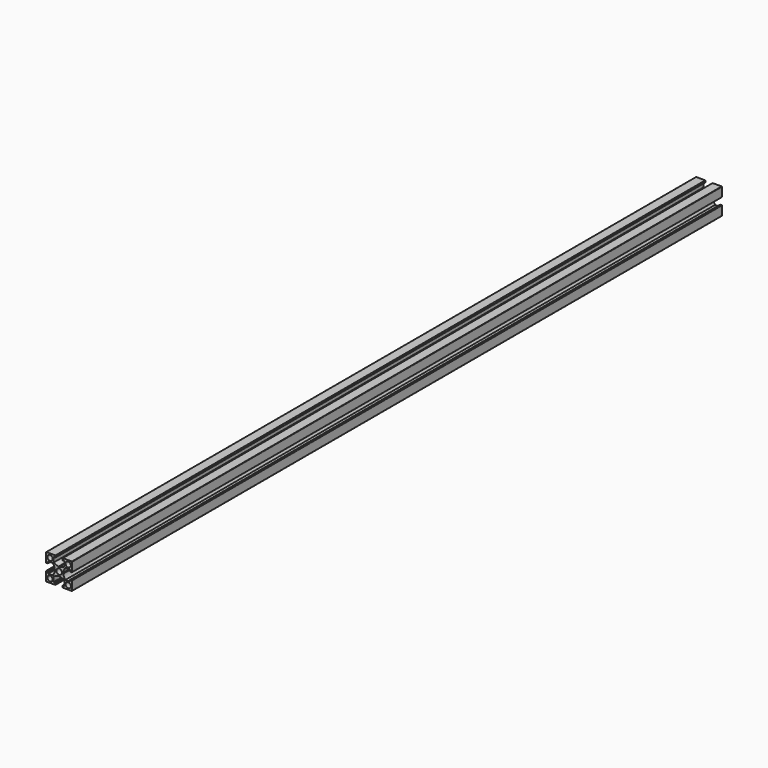
from build123d import *

# Parameters (mm, degrees)
F0_R     = 2
F0_R_2   = 2.15
F1_DEPTH = 312


# Not quite as in the source:
# - ends of sketch curves that miss each other by under 0.0002 mm in the source are joined


with BuildPart() as f1:
    # F0 (on Front) → F1 (new body, symmetric)
    with BuildSketch(Plane.XZ):
        with BuildLine():
            Line((4.49119, 14.509531), (4.49119, 11.252281))
            ThreePointArc((4.49119, 11.252281), (4.4613472004, 11.1218391084), (4.377756086, 11.0173488916))
            ThreePointArc((4.377756086, 11.0173488916), (2.6232116259, 10.0239112371), (0.6484679813, 9.6168093955))
            Line((0.6484679813, 9.6168093955), (0.34119, 9.309531))
            Line((0.34119, 9.309531), (0.033913, 9.616809))
            ThreePointArc((0.033913, 9.616809), (-1.9408311583, 10.0239110615), (-3.695375823, 11.0173492229))
            ThreePointArc((-3.695375823, 11.0173492229), (-3.7789672004, 11.1218391084), (-3.80881, 11.252281))
            Line((-3.80881, 11.252281), (-3.80881, 14.509531))
            ThreePointArc((-3.80881, 14.509531), (-3.7209420344, 14.7216630344), (-3.50881, 14.809531))
            Line((-3.50881, 14.809531), (-2.60881, 14.809531))
            ThreePointArc((-2.60881, 14.809531), (-2.3966779656, 14.8973989656), (-2.30881, 15.109531))
            Line((-2.30881, 15.109531), (-2.30881, 16.009531))
            ThreePointArc((-2.30881, 16.009531), (-2.3966779656, 16.2216630344), (-2.60881, 16.309531))
            Line((-2.60881, 16.309531), (-9.35881, 16.309531))
            ThreePointArc((-9.35881, 16.309531), (-9.5709420344, 16.2216630344), (-9.65881, 16.009531))
            Line((-9.65881, 16.009531), (-9.65881, 9.259531))
            ThreePointArc((-9.65881, 9.259531), (-9.5709420344, 9.0473989656), (-9.35881, 8.959531))
            Line((-9.35881, 8.959531), (-8.45881, 8.959531))
            ThreePointArc((-8.45881, 8.959531), (-8.2466779656, 9.0473989656), (-8.15881, 9.259531))
            Line((-8.15881, 9.259531), (-8.15881, 10.159531))
            ThreePointArc((-8.15881, 10.159531), (-8.0709420344, 10.3716630344), (-7.85881, 10.459531))
            Line((-7.85881, 10.459531), (-4.601559, 10.459531))
            ThreePointArc((-4.601559, 10.459531), (-4.471117461, 10.4296883706), (-4.3666273786, 10.3460976993))
            ThreePointArc((-4.3666273786, 10.3460976993), (-3.3731893747, 8.5915529924), (-2.9660873955, 6.6168089813))
            Line((-2.9660873955, 6.6168089813), (-2.65881, 6.309531))
            Line((-2.65881, 6.309531), (-2.966087, 6.002254))
            ThreePointArc((-2.966087, 6.002254), (-3.3731890615, 4.0275098417), (-4.3666272229, 2.272965177))
            ThreePointArc((-4.3666272229, 2.272965177), (-4.4711171084, 2.1893737996), (-4.601559, 2.159531))
            Line((-4.601559, 2.159531), (-7.85881, 2.159531))
            ThreePointArc((-7.85881, 2.159531), (-8.0709420344, 2.2473989656), (-8.15881, 2.459531))
            Line((-8.15881, 2.459531), (-8.15881, 3.359531))
            ThreePointArc((-8.15881, 3.359531), (-8.2466779656, 3.5716630344), (-8.45881, 3.659531))
            Line((-8.45881, 3.659531), (-9.35881, 3.659531))
            ThreePointArc((-9.35881, 3.659531), (-9.5709420344, 3.5716630344), (-9.65881, 3.359531))
            Line((-9.65881, 3.359531), (-9.65881, -3.390469))
            ThreePointArc((-9.65881, -3.390469), (-9.5709420344, -3.6026010344), (-9.35881, -3.690469))
            Line((-9.35881, -3.690469), (-2.60881, -3.690469))
            ThreePointArc((-2.60881, -3.690469), (-2.3966779656, -3.6026010344), (-2.30881, -3.390469))
            Line((-2.30881, -3.390469), (-2.30881, -2.490469))
            ThreePointArc((-2.30881, -2.490469), (-2.3966779656, -2.2783369656), (-2.60881, -2.190469))
            Line((-2.60881, -2.190469), (-3.50881, -2.190469))
            ThreePointArc((-3.50881, -2.190469), (-3.7209420344, -2.1026010344), (-3.80881, -1.890469))
            Line((-3.80881, -1.890469), (-3.80881, 1.366782))
            ThreePointArc((-3.80881, 1.366782), (-3.7789672004, 1.4972238916), (-3.695376086, 1.6017141084))
            ThreePointArc((-3.695376086, 1.6017141084), (-1.9408311583, 2.5951519385), (0.0339130165, 3.0022536517))
            Line((0.0339130165, 3.0022536517), (0.34119, 3.309531))
            Line((0.34119, 3.309531), (0.648468, 3.002254))
            ThreePointArc((0.648468, 3.002254), (2.6232116259, 2.5951517629), (4.377755823, 1.6017137771))
            ThreePointArc((4.377755823, 1.6017137771), (4.4613472004, 1.4972238916), (4.49119, 1.366782))
            Line((4.49119, 1.366782), (4.49119, -1.890469))
            ThreePointArc((4.49119, -1.890469), (4.4033220344, -2.1026010344), (4.19119, -2.190469))
            Line((4.19119, -2.190469), (3.29119, -2.190469))
            ThreePointArc((3.29119, -2.190469), (3.0790579656, -2.2783369656), (2.99119, -2.490469))
            Line((2.99119, -2.490469), (2.99119, -3.390469))
            ThreePointArc((2.99119, -3.390469), (3.0790579656, -3.6026010344), (3.29119, -3.690469))
            Line((3.29119, -3.690469), (10.04119, -3.690469))
            ThreePointArc((10.04119, -3.690469), (10.2533220344, -3.6026010344), (10.34119, -3.390469))
            Line((10.34119, -3.390469), (10.34119, 3.359531))
            ThreePointArc((10.34119, 3.359531), (10.2533220344, 3.5716630344), (10.04119, 3.659531))
            Line((10.04119, 3.659531), (9.14119, 3.659531))
            ThreePointArc((9.14119, 3.659531), (8.9290579656, 3.5716630344), (8.84119, 3.359531))
            Line((8.84119, 3.359531), (8.84119, 2.459531))
            ThreePointArc((8.84119, 2.459531), (8.7533220344, 2.2473989656), (8.54119, 2.159531))
            Line((8.54119, 2.159531), (5.28394, 2.159531))
            ThreePointArc((5.28394, 2.159531), (5.1534981084, 2.1893737996), (5.0490078916, 2.272964914))
            ThreePointArc((5.0490078916, 2.272964914), (4.0555700615, 4.0275098417), (3.6484683483, 6.0022540165))
            Line((3.6484683483, 6.0022540165), (3.34119, 6.309531))
            Line((3.34119, 6.309531), (3.648468, 6.616809))
            ThreePointArc((3.648468, 6.616809), (4.0555703747, 8.5915529924), (5.0490087099, 10.3460974363))
            ThreePointArc((5.0490087099, 10.3460974363), (5.153498461, 10.4296883706), (5.28394, 10.459531))
            Line((5.28394, 10.459531), (8.54119, 10.459531))
            ThreePointArc((8.54119, 10.459531), (8.7533220344, 10.3716630344), (8.84119, 10.159531))
            Line((8.84119, 10.159531), (8.84119, 9.259531))
            ThreePointArc((8.84119, 9.259531), (8.9290579656, 9.0473989656), (9.14119, 8.959531))
            Line((9.14119, 8.959531), (10.04119, 8.959531))
            ThreePointArc((10.04119, 8.959531), (10.2533220344, 9.0473989656), (10.34119, 9.259531))
            Line((10.34119, 9.259531), (10.34119, 16.009531))
            ThreePointArc((10.34119, 16.009531), (10.2533220344, 16.2216630344), (10.04119, 16.309531))
            Line((10.04119, 16.309531), (3.29119, 16.309531))
            ThreePointArc((3.29119, 16.309531), (3.0790579656, 16.2216630344), (2.99119, 16.009531))
            Line((2.99119, 16.009531), (2.99119, 15.109531))
            ThreePointArc((2.99119, 15.109531), (3.0790579656, 14.8973989656), (3.29119, 14.809531))
            Line((3.29119, 14.809531), (4.19119, 14.809531))
            ThreePointArc((4.19119, 14.809531), (4.4033220344, 14.7216630344), (4.49119, 14.509531))
        make_face()
        with Locations((-6.65881, -0.690469)):
            Circle(F0_R, mode=Mode.SUBTRACT)
        with Locations((7.34119, -0.690469)):
            Circle(F0_R, mode=Mode.SUBTRACT)
        with Locations((-6.65881, 13.309531)):
            Circle(F0_R, mode=Mode.SUBTRACT)
        with Locations((0.34119, 6.309531)):
            Circle(F0_R_2, mode=Mode.SUBTRACT)
        with Locations((7.34119, 13.309531)):
            Circle(F0_R, mode=Mode.SUBTRACT)
    extrude(amount=F1_DEPTH, both=True)


solid = f1.part
